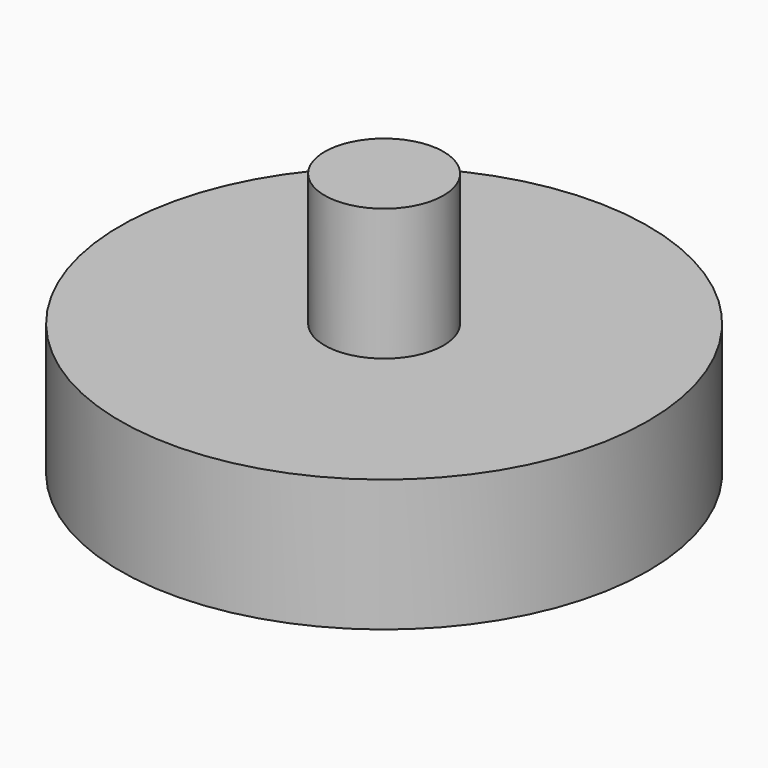
from build123d import *

# Parameters (mm, degrees)
F0_R     = 2.286
F1_DEPTH = 5.08
F2_R     = 10.16
F2_R_2   = 2.286
F3_DEPTH = 5.08


with BuildPart() as f1:
    # F0 (on Top) → F1 (new body)
    with BuildSketch(Plane.XY):
        Circle(F0_R)
    extrude(amount=F1_DEPTH)

    # F2 (on face) → F3 (join)
    with BuildSketch(Plane(origin=(0, 0, 0), x_dir=(1, 0, 0), z_dir=(0, 0, -1))):
        Circle(F2_R)
        Circle(F2_R_2, mode=Mode.SUBTRACT)
        Circle(F2_R_2)
    extrude(amount=F3_DEPTH)


solid = f1.part
